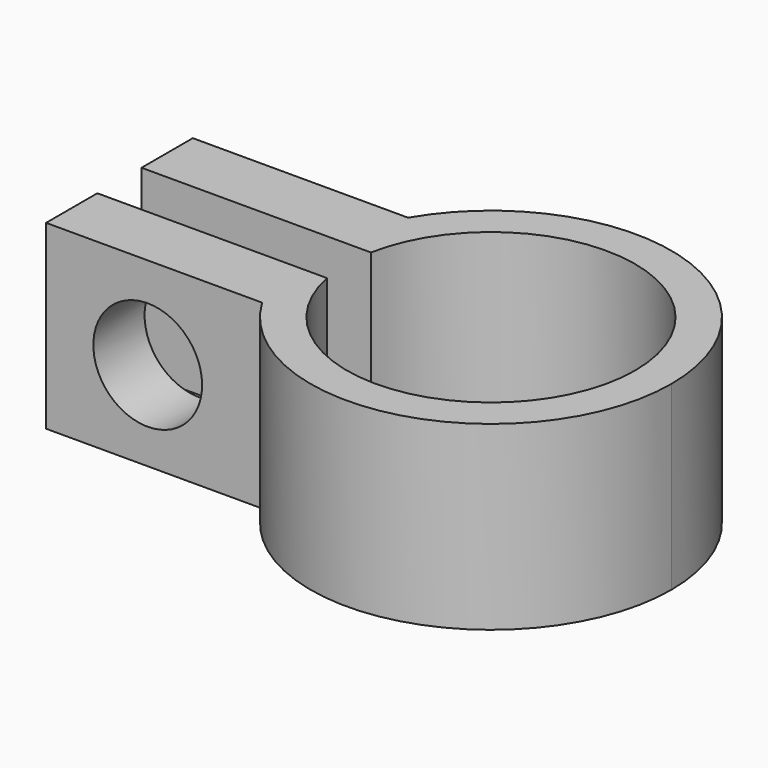
from build123d import *

# Parameters (mm, degrees)
F1_DEPTH = 5
F2_R     = 1.5
F3_DEPTH = 25.4


with BuildPart() as f1:
    # F0 (on Top) → F1 (new body)
    with BuildSketch(Plane.XY):
        with BuildLine():
            Line((-10.2344341576, 0.7447922041), (-4.9204421579, 0.7447922041))
            ThreePointArc((-4.9204421579, 0.7447922041), (-4.6921521255, 1.6580635959), (-4.2959631379, 2.5120046127))
            Line((-4.2959631379, 2.5120046127), (-10.2344341576, 2.5120046127))
            Line((-10.2344341576, 2.5120046127), (-10.2344341576, 0.7447922041))
        make_face()
        with BuildLine():
            ThreePointArc((-4.2756532365, -2.5464202045), (-4.6795608737, -1.6932738958), (-4.9151095275, -0.7792077959))
            Line((-4.9151095275, -0.7792077959), (-10.2344341576, -0.7792077959))
            Line((-10.2344341576, -0.7792077959), (-10.2344341576, -2.5464202045))
            Line((-10.2344341576, -2.5464202045), (-4.2756532365, -2.5464202045))
        make_face()
        with BuildLine():
            ThreePointArc((-3.9061193363, 0.7447922041), (0.3740546925, 3.9588592781), (3.9764913802, 0))
            ThreePointArc((3.9764913802, 0), (0.391506034, -3.9571715558), (-3.8993998137, -0.7792077959))
            Line((-3.8993998137, -0.7792077959), (-4.9151095275, -0.7792077959))
            ThreePointArc((-4.9151095275, -0.7792077959), (-4.6795608737, -1.6932738958), (-4.2756532365, -2.5464202045))
            ThreePointArc((-4.2756532365, -2.5464202045), (1.3205519643, -4.7980838849), (4.9764913802, 0))
            ThreePointArc((4.9764913802, 0), (1.3012768598, 4.8033472695), (-4.2959631379, 2.5120046127))
            ThreePointArc((-4.2959631379, 2.5120046127), (-4.6921521255, 1.6580635959), (-4.9204421579, 0.7447922041))
            Line((-4.9204421579, 0.7447922041), (-3.9061193363, 0.7447922041))
        make_face()
    extrude(amount=F1_DEPTH)

    # F2 (on face) → F3 (cut)
    with BuildSketch(Plane.XZ.offset(2.5464202045)):
        with Locations((-7.4309720658, 2.4591526017)):
            Circle(F2_R)
    extrude(amount=-F3_DEPTH, mode=Mode.SUBTRACT)


solid = f1.part
